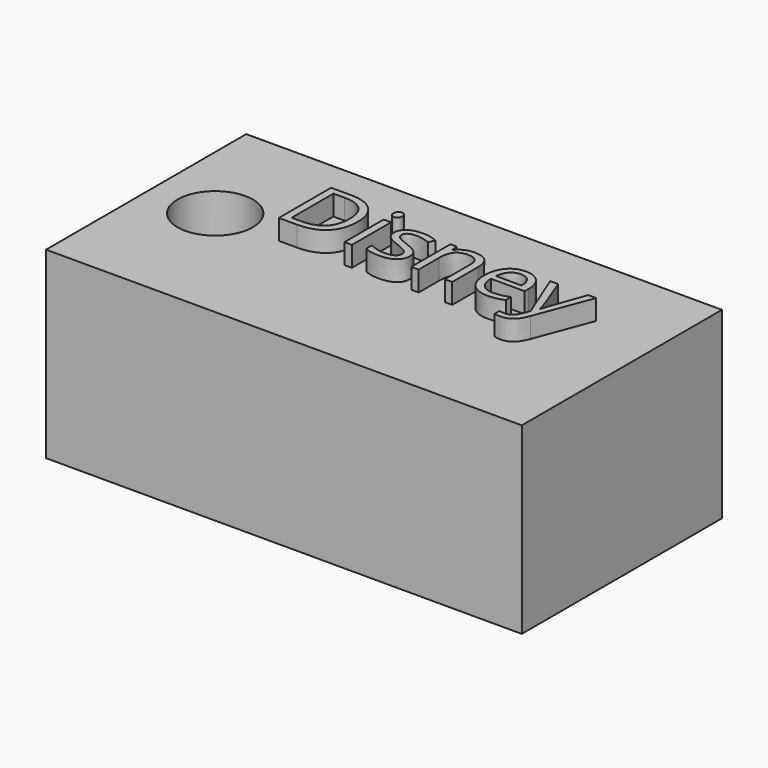
from build123d import *

# Parameters (mm, degrees)
F0_W         = 65.8026188612
F0_H         = 34.6104670316
F1_DEPTH     = 25.4
F2_R         = 5.2107749701
F3_DEPTH     = 25.4
F4_TEXT_SIZE = 12.6622824205
F5_DEPTH     = 2.794


# Not quite as in the source:
# - Text() gives the source's letters only with a copy of the font that has no kerning and outlines rounded to 1/6400 em; it was checked with that copy


with BuildPart() as f1:
    # F0 (on Top) → F1 (new body)
    with BuildSketch(Plane.XY):
        with Locations((-50.9543009102, 28.2011218369)):
            Rectangle(F0_W, F0_H)
    extrude(amount=F1_DEPTH)

    # F2 (on face) → F3 (cut)
    with BuildSketch(Plane.XY.offset(25.4)):
        with Locations((-74.8890563846, 28.9288982749)):
            Circle(F2_R)
    extrude(amount=-F3_DEPTH, mode=Mode.SUBTRACT)

    # F4 (on face) → F5 (join)
    with BuildSketch(Plane.XY.offset(25.4)):
        with Locations((-66.7466074228, 28.2011218369)):
            Text('Disney', F4_TEXT_SIZE, font='Open Sans', text_align=(TextAlign.LEFT, TextAlign.BOTTOM))
    extrude(amount=F5_DEPTH)


solid = f1.part
